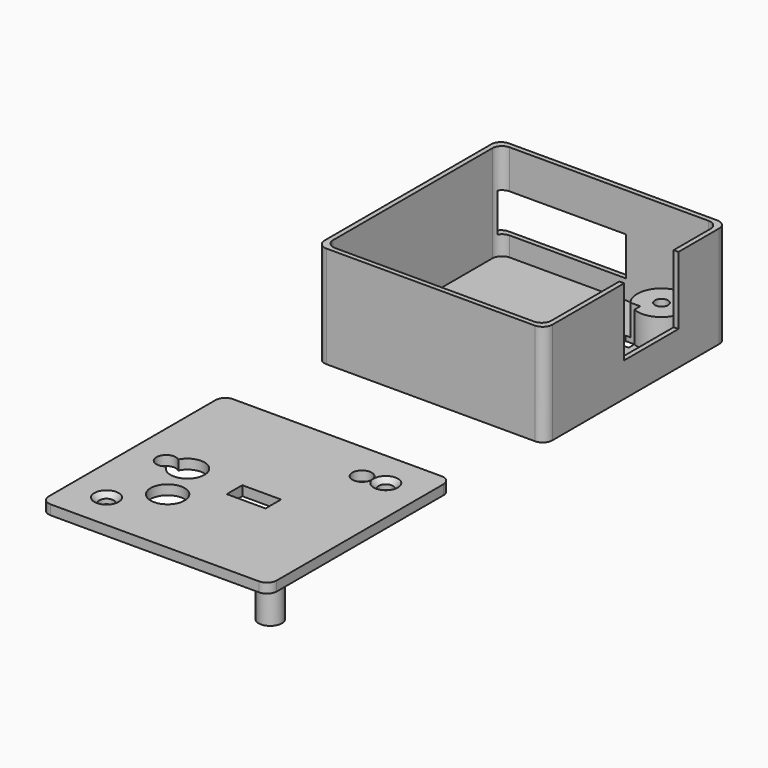
from build123d import *

# Parameters (mm, degrees)
F0_W      = 47
F0_H      = 47
F1_DEPTH  = 21
F2_W      = 45
F2_H      = 45
F3_DEPTH  = 20
F5_R      = 2.5
F5_R_2    = 1.35
F6_DEPTH  = 6.3
F7_DEPTH  = 2
F8_R      = 5
F8_R_2    = 2.5
F9_DEPTH  = 6.3
F10_R     = 1.35
F11_DEPTH = 2
F12_W     = 47
F12_H     = 47
F12_R     = 1.5
F12_R_2   = 2.5
F13_DEPTH = 2
F14_SIZE  = 1
F15_R     = 2
F16_R     = 2
F17_W     = 25
F17_H     = 8
F17_W_2   = 2
F18_DEPTH = 2
F19_W     = 14
F19_H     = 14
F20_DEPTH = 3
F21_R     = 3.5
F21_R_2   = 2
F21_W     = 8
F21_H     = 4
F22_DEPTH = 5
F23_R     = 4.5
F23_W     = 3
F23_H     = 3
F24_DEPTH = 10
F25_R     = 2.3636646969
F25_R_2   = 2.3886353596
F26_DEPTH = 10.8


with BuildPart() as f1:
    # F0 (on Top) → F1 (new body)
    with BuildSketch(Plane.XY):
        with Locations((-36.5994639099, 36.4211554304)):
            Rectangle(F0_W, F0_H)
    extrude(amount=F1_DEPTH)

    # F2 (on face) → F3 (cut)
    with BuildSketch(Plane.XY.offset(21)):
        with Locations((-36.5994639099, 36.4211554304)):
            Rectangle(F2_W, F2_H)
    extrude(amount=-F3_DEPTH, mode=Mode.SUBTRACT)

    # F5 (on face) → F6 (join)
    with BuildSketch(Plane.XY.offset(1)):
        with Locations((-52.5994639099, 20.4211554304)):
            Circle(F5_R)
        with Locations((-52.5994639099, 20.4211554304)):
            Circle(F5_R_2, mode=Mode.SUBTRACT)
        with Locations((-20.5994639099, 52.4211554304)):
            Circle(F5_R)
        with Locations((-20.5994639099, 52.4211554304)):
            Circle(F5_R_2, mode=Mode.SUBTRACT)
    extrude(amount=F6_DEPTH)

    # F7 (cut): faces of the model
    f7_faces = [f1.faces().sort_by_distance(p)[0] for p in [
        (-52.5994639099, 20.4211554304, 1),
        (-20.5994639099, 52.4211554304, 1),
    ]]
    extrude(f7_faces, amount=-F7_DEPTH, mode=Mode.SUBTRACT)

    # F8 (on face) → F9 (join)
    with BuildSketch(Plane.XY.offset(1)):
        with Locations((-52.5994639099, 20.4211554304)):
            Circle(F8_R)
        with Locations((-52.5994639099, 20.4211554304)):
            Circle(F8_R_2, mode=Mode.SUBTRACT)
        with Locations((-20.5994639099, 52.4211554304)):
            Circle(F8_R)
        with Locations((-20.5994639099, 52.4211554304)):
            Circle(F8_R_2, mode=Mode.SUBTRACT)
    extrude(amount=F9_DEPTH)

    # F10 (on face) → F11 (cut)
    with BuildSketch(Plane(origin=(0, 0, 0), x_dir=(1, 0, 0), z_dir=(0, 0, -1))):
        Polygon((-49.5999728624, -20.4764135179), (-51.0518634785, -17.8511490286), (-54.051354526, -17.7958909411), (-55.5989549573, -20.3658973428), (-54.1470643412, -22.9911618321), (-51.1475732937, -23.0464199197), align=None)
        with Locations((-52.5994639099, -20.4211554304)):
            Circle(F10_R, mode=Mode.SUBTRACT)
        Polygon((-18.7069320828, -54.7488846422), (-17.6373253658, -51.9460393966), (-19.5298571928, -49.6183101848), (-22.4919957369, -50.0934262185), (-23.561602454, -52.8962714641), (-21.669070627, -55.224000676), align=None)
        with Locations((-20.5994639099, -52.4211554304)):
            Circle(F10_R, mode=Mode.SUBTRACT)
    extrude(amount=-F11_DEPTH, mode=Mode.SUBTRACT)

    # F16
    f16_edges = [f1.edges().sort_by_distance(p)[0] for p in [
        (-60.099464, 12.921155, 10.5),
        (-13.099464, 59.921155, 10.5),
        (-13.099464, 12.921155, 10.5),
        (-59.099464, 13.921155, 11),
        (-14.099464, 13.921155, 11),
        (-59.099464, 58.921155, 11),
        (-14.099464, 58.921155, 11),
        (-60.099464, 59.921155, 10.5),
    ]]
    fillet(f16_edges, radius=F16_R)

    # F17 (on face) → F18 (cut)
    with BuildSketch(Plane(origin=(0, 59.9211554304, 0), x_dir=(-1, 0, 0), z_dir=(0, 1, 0))):
        with Locations((45.5994639099, 9)):
            Rectangle(F17_W, F17_H)
        with Locations((59.0994639099, 9)):
            Rectangle(F17_W_2, F17_H)
    extrude(amount=-F18_DEPTH, mode=Mode.SUBTRACT)

    # F19 (on face) → F20 (cut)
    with BuildSketch(Plane.YZ.offset(-13.0994639099)):
        with Locations((40.4211554304, 14)):
            Rectangle(F19_W, F19_H)
    extrude(amount=-F20_DEPTH, mode=Mode.SUBTRACT)

    # F23 (on face) → F24 (cut)
    with BuildSketch(Plane(origin=(0, 0, 0), x_dir=(1, 0, 0), z_dir=(0, 0, -1))):
        with Locations((-37.5994639099, -24.9211554304)):
            Circle(F23_R)
        with Locations((-23.9994639099, -47.8211554304)):
            Rectangle(F23_W, F23_H)
    extrude(amount=-F24_DEPTH, mode=Mode.SUBTRACT)


with BuildPart() as f13:
    # F12 (on Top) → F13 (new body)
    with BuildSketch(Plane.XY):
        with Locations((-38.3334934391, -32.4880076721)):
            Rectangle(F12_W, F12_H)
        with Locations((-58.3334934391, -52.4880076721)):
            Circle(F12_R, mode=Mode.SUBTRACT)
        with Locations((-54.3334934391, -48.4880076721)):
            Circle(F12_R_2, mode=Mode.SUBTRACT)
        with Locations((-18.3334934391, -52.4880076721)):
            Circle(F12_R, mode=Mode.SUBTRACT)
        with Locations((-58.3334934391, -12.4880076721)):
            Circle(F12_R, mode=Mode.SUBTRACT)
        with Locations((-22.3334934391, -16.4880076721)):
            Circle(F12_R_2, mode=Mode.SUBTRACT)
        with Locations((-18.3334934391, -12.4880076721)):
            Circle(F12_R, mode=Mode.SUBTRACT)
        with Locations((-58.3334934391, -12.4880076721)):
            Circle(F12_R)
        with Locations((-18.3334934391, -12.4880076721)):
            Circle(F12_R)
        with Locations((-18.3334934391, -52.4880076721)):
            Circle(F12_R)
        with Locations((-58.3334934391, -52.4880076721)):
            Circle(F12_R)
        with Locations((-22.3334934391, -16.4880076721)):
            Circle(F12_R_2)
        with Locations((-22.3334934391, -16.4880076721)):
            Circle(F12_R, mode=Mode.SUBTRACT)
        with Locations((-54.3334934391, -48.4880076721)):
            Circle(F12_R_2)
        with Locations((-54.3334934391, -48.4880076721)):
            Circle(F12_R, mode=Mode.SUBTRACT)
    extrude(amount=F13_DEPTH)

    # F14
    f14_edges = [f13.edges().sort_by_distance(p)[0] for p in [
        (-23.833493, -16.488008, 2),
        (-55.833493, -48.488008, 2),
    ]]
    chamfer(f14_edges, length=F14_SIZE)

    # F15
    f15_edges = [f13.edges().sort_by_distance(p)[0] for p in [
        (-61.833493, -55.988008, 1),
        (-61.833493, -8.988008, 1),
        (-14.833493, -8.988008, 1),
        (-14.833493, -55.988008, 1),
    ]]
    fillet(f15_edges, radius=F15_R)

    # F21 (on face) → F22 (cut)
    with BuildSketch(Plane.XY.offset(2)):
        with Locations((-47.3334934391, -41.4880076721)):
            Circle(F21_R)
        with Locations((-26.8334934391, -16.9880076721)):
            Circle(F21_R_2)
        with Locations((-35.9334934391, -33.4880076721)):
            Rectangle(F21_W, F21_H)
        with BuildLine():
            ThreePointArc((-53.5709934391, -34.0391665131), (-49.637016823, -35.8961780024), (-46.9334934391, -32.4880076721))
            ThreePointArc((-46.9334934391, -32.4880076721), (-49.637016823, -29.0798373419), (-53.5709934391, -30.9368488311))
            ThreePointArc((-53.5709934391, -30.9368488311), (-53.0272542523, -31.6292294703), (-52.8334934391, -32.4880076721))
            ThreePointArc((-52.8334934391, -32.4880076721), (-53.0272542523, -33.346785874), (-53.5709934391, -34.0391665131))
        make_face()
        with BuildLine():
            ThreePointArc((-52.8334934391, -32.4880076721), (-53.0272542523, -31.6292294703), (-53.5709934391, -30.9368488311))
            ThreePointArc((-53.5709934391, -30.9368488311), (-53.9334934391, -32.4880076721), (-53.5709934391, -34.0391665131))
            ThreePointArc((-53.5709934391, -34.0391665131), (-53.0272542523, -33.346785874), (-52.8334934391, -32.4880076721))
        make_face()
        with BuildLine():
            ThreePointArc((-53.5709934391, -34.0391665131), (-53.9334934391, -32.4880076721), (-53.5709934391, -30.9368488311))
            ThreePointArc((-53.5709934391, -30.9368488311), (-56.8334934391, -32.4880076721), (-53.5709934391, -34.0391665131))
        make_face()
    extrude(amount=-F22_DEPTH, mode=Mode.SUBTRACT)

    # F25 (on face) → F26 (join)
    with BuildSketch(Plane(origin=(0, 0, 0), x_dir=(1, 0, 0), z_dir=(0, 0, -1))):
        with Locations((-49.9348416924, 23.4782043844)):
            Circle(F25_R)
        with Locations((-22.6007383317, 45.9453836083)):
            Circle(F25_R_2)
    extrude(amount=F26_DEPTH)


solid = Compound([f1.part, f13.part])
